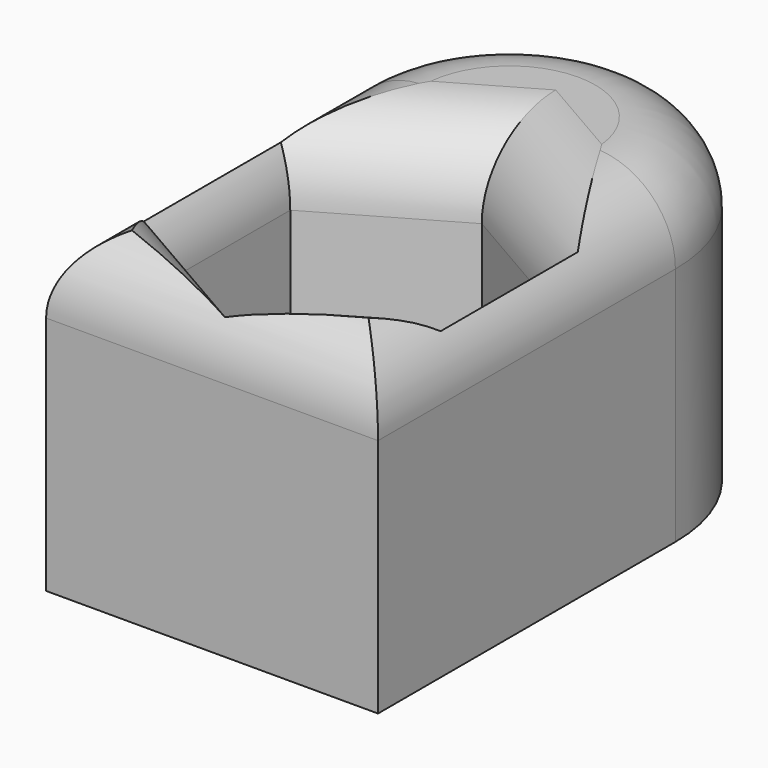
from build123d import *

# Parameters (mm, degrees)
F1_DEPTH      = 50.8
F2_T1_DEPTH   = 58.9474439621
F2_T3_DEPTH   = 52.6393949986
F2_T6_ANGLE   = 180
F2_T10_DEPTH  = 87.4865868528
F2_T16_DEPTH  = 87.4865868528
F2_T22_DEPTH  = 87.4865868528
F2_T28_DEPTH  = 87.4865868528
F2_T34_DEPTH  = 87.4865868528
F2_T40_DEPTH  = 87.4865868528
F2_T47_DEPTH  = 90.6974439621
F2_T51_DEPTH  = 84.3893949986
F2_T58_DEPTH  = 84.3893949986
F2_T62_DEPTH  = 90.6974439621
F2_T69_DEPTH  = 87.4865868528
F2_T73_DEPTH  = 87.4865868528
F2_T80_DEPTH  = 87.4865868528
F2_T84_DEPTH  = 87.4865868528
F2_T91_DEPTH  = 87.4865868528
F2_T95_DEPTH  = 87.4865868528
F2_T102_DEPTH = 87.4865868528
F2_T106_DEPTH = 87.4865868528
F2_T113_DEPTH = 87.4865868528
F2_T117_DEPTH = 87.4865868528
F2_T124_DEPTH = 87.4865868528
F2_T128_DEPTH = 87.4865868528


# Not quite as in the source:
# - a fillet or chamfer that OpenCascade refuses, or shapes differently, is made with other operations: its cross-section is extruded or revolved along the edge and cut away or added
# - a feature names something its author has since deleted; it is built from what else it names


with BuildPart() as f1:
    # F0 (on Top) → F1 (new body)
    with BuildSketch(Plane.XY):
        with BuildLine():
            Line((-26.3196974993, -29.473721981), (26.3196974993, -29.473721981))
            Line((26.3196974993, -29.473721981), (26.3196974993, 29.473721981))
            ThreePointArc((26.3196974993, 29.473721981), (0, 55.7934194803), (-26.3196974993, 29.473721981))
            Line((-26.3196974993, 29.473721981), (-26.3196974993, -29.473721981))
        make_face()
        Polygon((0, 23.9865868528), (20.7729935646, 11.9932934264), (20.7729935646, -11.9932934264), (0, -23.9865868528), (-20.7729935646, -11.9932934264), (-20.7729935646, 11.9932934264), align=None, mode=Mode.SUBTRACT)
    extrude(amount=F1_DEPTH)

    # F2: fillet of radius 12.7 on 10 edges, made by hand

    # F2_s2 → F2_t1 (cut)
    with BuildSketch(Plane.XZ.offset(-29.473721981)):
        with BuildLine():
            ThreePointArc((-26.3196974993, 38.1), (-22.5999536203, 47.0802561211), (-13.6196974993, 50.8))
            Line((-13.6196974993, 50.8), (-13.6196974993, 51.054))
            Line((-13.6196974993, 51.054), (-26.5736974993, 51.054))
            Line((-26.5736974993, 51.054), (-26.5736974993, 38.1))
            Line((-26.5736974993, 38.1), (-26.3196974993, 38.1))
        make_face()
        with BuildLine():
            ThreePointArc((26.3196974993, 38.1), (22.5999536203, 47.0802561211), (13.6196974993, 50.8))
            Line((13.6196974993, 50.8), (13.6196974993, 51.054))
            Line((13.6196974993, 51.054), (26.5736974993, 51.054))
            Line((26.5736974993, 51.054), (26.5736974993, 38.1))
            Line((26.5736974993, 38.1), (26.3196974993, 38.1))
        make_face()
    extrude(amount=F2_T1_DEPTH, mode=Mode.SUBTRACT)

    # F2_s4 → F2_t3 (cut)
    with BuildSketch(Plane.YZ.offset(-26.3196974993)):
        with BuildLine():
            ThreePointArc((-29.473721981, 38.1), (-25.7539781021, 47.0802561211), (-16.773721981, 50.8))
            Line((-16.773721981, 50.8), (-16.773721981, 51.054))
            Line((-16.773721981, 51.054), (-29.727721981, 51.054))
            Line((-29.727721981, 51.054), (-29.727721981, 38.1))
            Line((-29.727721981, 38.1), (-29.473721981, 38.1))
        make_face()
    extrude(amount=F2_T3_DEPTH, mode=Mode.SUBTRACT)

    # F2_s5 → F2_t6 (revolve, cut)
    with BuildSketch(Plane.XZ.offset(-29.473721981)):
        with BuildLine():
            ThreePointArc((26.3196974993, 38.1), (22.5999536203, 47.0802561211), (13.6196974993, 50.8))
            Line((13.6196974993, 50.8), (13.6196974993, 51.054))
            Line((13.6196974993, 51.054), (26.5736974993, 51.054))
            Line((26.5736974993, 51.054), (26.5736974993, 38.1))
            Line((26.5736974993, 38.1), (26.3196974993, 38.1))
        make_face()
    revolve(axis=Axis((0, 29.473721981, 50.8), (0, 0, 1)), revolution_arc=F2_T6_ANGLE, mode=Mode.SUBTRACT)


with BuildPart() as f2_tool8:
    # F2_s9 → F2_t10 (new body)
    with BuildSketch(Plane(origin=(-37.8828033525, -21.8716467132, 0), x_dir=(0, 0, 1), z_dir=(0.8660254038, 0.5, 0))):
        with BuildLine():
            ThreePointArc((38.1, -20.7729935646), (47.0802561211, -24.4927374435), (50.8, -33.4729935646))
            Line((50.8, -33.4729935646), (51.054, -33.4729935646))
            Line((51.054, -33.4729935646), (51.054, -20.5189935646))
            Line((51.054, -20.5189935646), (38.1, -20.5189935646))
            Line((38.1, -20.5189935646), (38.1, -20.7729935646))
        make_face()
    extrude(amount=F2_T10_DEPTH)

    split(bisect_by=Plane.YZ.offset(-20.7729935646), keep=Keep.TOP)

    split(bisect_by=Plane(origin=(10.3864967823, 17.9899401396, 0), x_dir=(0, 0, 1), z_dir=(-0.5, -0.8660254038, 0)), keep=Keep.TOP)


with BuildPart() as f1_1:
    add(f1.part)

    # F2_t7: cut F2_tool8
    add(f2_tool8.part, mode=Mode.SUBTRACT)


with BuildPart() as f2_tool14:
    # F2_s15 → F2_t16 (new body)
    with BuildSketch(Plane(origin=(-37.8828033525, 21.8716467132, 0), x_dir=(0, 0, 1), z_dir=(0.8660254038, -0.5, 0))):
        with BuildLine():
            ThreePointArc((38.1, -20.7729935646), (47.0802561211, -24.4927374435), (50.8, -33.4729935646))
            Line((50.8, -33.4729935646), (51.054, -33.4729935646))
            Line((51.054, -33.4729935646), (51.054, -20.5189935646))
            Line((51.054, -20.5189935646), (38.1, -20.5189935646))
            Line((38.1, -20.5189935646), (38.1, -20.7729935646))
        make_face()
    extrude(amount=F2_T16_DEPTH)

    split(bisect_by=Plane(origin=(-10.3864967823, 17.9899401396, 0), x_dir=(0, 0, 1), z_dir=(0.5, -0.8660254038, 0)), keep=Keep.TOP)

    split(bisect_by=Plane.YZ.offset(20.7729935646), keep=Keep.BOTTOM)


with BuildPart() as f1_2:
    add(f1_1.part)

    # F2_t13: cut F2_tool14
    add(f2_tool14.part, mode=Mode.SUBTRACT)


with BuildPart() as f2_tool20:
    # F2_s21 → F2_t22 (new body)
    with BuildSketch(Plane.XZ.offset(-43.7432934264)):
        with BuildLine():
            ThreePointArc((20.7729935646, 38.1), (24.4927374435, 47.0802561211), (33.4729935646, 50.8))
            Line((33.4729935646, 50.8), (33.4729935646, 51.054))
            Line((33.4729935646, 51.054), (20.5189935646, 51.054))
            Line((20.5189935646, 51.054), (20.5189935646, 38.1))
            Line((20.5189935646, 38.1), (20.7729935646, 38.1))
        make_face()
    extrude(amount=F2_T22_DEPTH)

    split(bisect_by=Plane(origin=(10.3864967823, 17.9899401396, 0), x_dir=(0, 0, 1), z_dir=(-0.5, -0.8660254038, 0)), keep=Keep.TOP)

    split(bisect_by=Plane(origin=(10.3864967823, -17.9899401396, 0), x_dir=(0, 0, 1), z_dir=(-0.5, 0.8660254038, 0)), keep=Keep.TOP)


with BuildPart() as f1_3:
    add(f1_2.part)

    # F2_t19: cut F2_tool20
    add(f2_tool20.part, mode=Mode.SUBTRACT)


with BuildPart() as f2_tool26:
    # F2_s27 → F2_t28 (new body)
    with BuildSketch(Plane(origin=(37.8828033525, 21.8716467132, 0), x_dir=(0, 0, 1), z_dir=(-0.8660254038, -0.5, 0))):
        with BuildLine():
            ThreePointArc((38.1, -20.7729935646), (47.0802561211, -24.4927374435), (50.8, -33.4729935646))
            Line((50.8, -33.4729935646), (51.054, -33.4729935646))
            Line((51.054, -33.4729935646), (51.054, -20.5189935646))
            Line((51.054, -20.5189935646), (38.1, -20.5189935646))
            Line((38.1, -20.5189935646), (38.1, -20.7729935646))
        make_face()
    extrude(amount=F2_T28_DEPTH)

    split(bisect_by=Plane.YZ.offset(20.7729935646), keep=Keep.BOTTOM)

    split(bisect_by=Plane(origin=(-10.3864967823, -17.9899401396, 0), x_dir=(0, 0, 1), z_dir=(0.5, 0.8660254038, 0)), keep=Keep.TOP)


with BuildPart() as f1_4:
    add(f1_3.part)

    # F2_t25: cut F2_tool26
    add(f2_tool26.part, mode=Mode.SUBTRACT)


with BuildPart() as f2_tool32:
    # F2_s33 → F2_t34 (new body)
    with BuildSketch(Plane(origin=(37.8828033525, -21.8716467132, 0), x_dir=(0, 0, 1), z_dir=(-0.8660254038, 0.5, 0))):
        with BuildLine():
            ThreePointArc((38.1, -20.7729935646), (47.0802561211, -24.4927374435), (50.8, -33.4729935646))
            Line((50.8, -33.4729935646), (51.054, -33.4729935646))
            Line((51.054, -33.4729935646), (51.054, -20.5189935646))
            Line((51.054, -20.5189935646), (38.1, -20.5189935646))
            Line((38.1, -20.5189935646), (38.1, -20.7729935646))
        make_face()
    extrude(amount=F2_T34_DEPTH)

    split(bisect_by=Plane(origin=(10.3864967823, -17.9899401396, 0), x_dir=(0, 0, 1), z_dir=(-0.5, 0.8660254038, 0)), keep=Keep.TOP)

    split(bisect_by=Plane.YZ.offset(-20.7729935646), keep=Keep.TOP)


with BuildPart() as f1_5:
    add(f1_4.part)

    # F2_t31: cut F2_tool32
    add(f2_tool32.part, mode=Mode.SUBTRACT)


with BuildPart() as f2_tool38:
    # F2_s39 → F2_t40 (new body)
    with BuildSketch(Plane.XZ.offset(43.7432934264)):
        with BuildLine():
            ThreePointArc((-20.7729935646, 38.1), (-24.4927374435, 47.0802561211), (-33.4729935646, 50.8))
            Line((-33.4729935646, 50.8), (-33.4729935646, 51.054))
            Line((-33.4729935646, 51.054), (-20.5189935646, 51.054))
            Line((-20.5189935646, 51.054), (-20.5189935646, 38.1))
            Line((-20.5189935646, 38.1), (-20.7729935646, 38.1))
        make_face()
    extrude(amount=-F2_T40_DEPTH)

    split(bisect_by=Plane(origin=(-10.3864967823, 17.9899401396, 0), x_dir=(0, 0, 1), z_dir=(0.5, -0.8660254038, 0)), keep=Keep.TOP)

    split(bisect_by=Plane(origin=(-10.3864967823, -17.9899401396, 0), x_dir=(0, 0, 1), z_dir=(0.5, 0.8660254038, 0)), keep=Keep.TOP)


with BuildPart() as f1_6:
    add(f1_5.part)

    # F2_t37: cut F2_tool38
    add(f2_tool38.part, mode=Mode.SUBTRACT)


with BuildPart() as f2_tool45:
    # F2_s46 → F2_t47 (new body)
    with BuildSketch(Plane.XZ.offset(-29.473721981)):
        with BuildLine():
            ThreePointArc((-26.3196974993, 38.1), (-22.5999536203, 47.0802561211), (-13.6196974993, 50.8))
            Line((-13.6196974993, 50.8), (-13.6196974993, 51.054))
            Line((-13.6196974993, 51.054), (-26.5736974993, 51.054))
            Line((-26.5736974993, 51.054), (-26.5736974993, 38.1))
            Line((-26.5736974993, 38.1), (-26.3196974993, 38.1))
        make_face()
    extrude(amount=F2_T47_DEPTH)

    split(bisect_by=Plane.XZ.offset(29.473721981), keep=Keep.TOP)


with BuildPart() as f2_tool49:
    # F2_s50 → F2_t51 (new body)
    with BuildSketch(Plane.YZ.offset(-58.0696974993)):
        with BuildLine():
            ThreePointArc((-29.473721981, 38.1), (-25.7539781021, 47.0802561211), (-16.773721981, 50.8))
            Line((-16.773721981, 50.8), (-16.773721981, 51.054))
            Line((-16.773721981, 51.054), (-29.727721981, 51.054))
            Line((-29.727721981, 51.054), (-29.727721981, 38.1))
            Line((-29.727721981, 38.1), (-29.473721981, 38.1))
        make_face()
    extrude(amount=F2_T51_DEPTH)

    split(bisect_by=Plane.YZ.offset(-26.3196974993), keep=Keep.BOTTOM)


with BuildPart() as f2_tool45_1:
    add(f2_tool45.part)

    # F2_t53: intersect F2_tool49
    add(f2_tool49.part, mode=Mode.INTERSECT)


with BuildPart() as f1_7:
    add(f1_6.part)

    # F2_t43: cut F2_tool45
    add(f2_tool45_1.part, mode=Mode.SUBTRACT)


with BuildPart() as f2_tool56:
    # F2_s57 → F2_t58 (new body)
    with BuildSketch(Plane.YZ.offset(-26.3196974993)):
        with BuildLine():
            ThreePointArc((-29.473721981, 38.1), (-25.7539781021, 47.0802561211), (-16.773721981, 50.8))
            Line((-16.773721981, 50.8), (-16.773721981, 51.054))
            Line((-16.773721981, 51.054), (-29.727721981, 51.054))
            Line((-29.727721981, 51.054), (-29.727721981, 38.1))
            Line((-29.727721981, 38.1), (-29.473721981, 38.1))
        make_face()
    extrude(amount=F2_T58_DEPTH)

    split(bisect_by=Plane.YZ.offset(26.3196974993), keep=Keep.TOP)


with BuildPart() as f2_tool60:
    # F2_s61 → F2_t62 (new body)
    with BuildSketch(Plane.XZ.offset(61.223721981)):
        with BuildLine():
            ThreePointArc((26.3196974993, 38.1), (22.5999536203, 47.0802561211), (13.6196974993, 50.8))
            Line((13.6196974993, 50.8), (13.6196974993, 51.054))
            Line((13.6196974993, 51.054), (26.5736974993, 51.054))
            Line((26.5736974993, 51.054), (26.5736974993, 38.1))
            Line((26.5736974993, 38.1), (26.3196974993, 38.1))
        make_face()
    extrude(amount=-F2_T62_DEPTH)

    split(bisect_by=Plane.XZ.offset(29.473721981), keep=Keep.TOP)


with BuildPart() as f2_tool56_1:
    add(f2_tool56.part)

    # F2_t64: intersect F2_tool60
    add(f2_tool60.part, mode=Mode.INTERSECT)


with BuildPart() as f1_8:
    add(f1_7.part)

    # F2_t54: cut F2_tool56
    add(f2_tool56_1.part, mode=Mode.SUBTRACT)


with BuildPart() as f2_tool67:
    # F2_s68 → F2_t69 (new body)
    with BuildSketch(Plane(origin=(-37.8828033525, -21.8716467132, 0), x_dir=(0, 0, 1), z_dir=(0.8660254038, 0.5, 0))):
        with BuildLine():
            ThreePointArc((38.1, -20.7729935646), (47.0802561211, -24.4927374435), (50.8, -33.4729935646))
            Line((50.8, -33.4729935646), (51.054, -33.4729935646))
            Line((51.054, -33.4729935646), (51.054, -20.5189935646))
            Line((51.054, -20.5189935646), (38.1, -20.5189935646))
            Line((38.1, -20.5189935646), (38.1, -20.7729935646))
        make_face()
    extrude(amount=F2_T69_DEPTH)

    split(bisect_by=Plane.YZ.offset(-20.7729935646), keep=Keep.BOTTOM)


with BuildPart() as f2_tool71:
    # F2_s72 → F2_t73 (new body)
    with BuildSketch(Plane.XZ.offset(43.7432934264)):
        with BuildLine():
            ThreePointArc((-20.7729935646, 38.1), (-24.4927374435, 47.0802561211), (-33.4729935646, 50.8))
            Line((-33.4729935646, 50.8), (-33.4729935646, 51.054))
            Line((-33.4729935646, 51.054), (-20.5189935646, 51.054))
            Line((-20.5189935646, 51.054), (-20.5189935646, 38.1))
            Line((-20.5189935646, 38.1), (-20.7729935646, 38.1))
        make_face()
    extrude(amount=-F2_T73_DEPTH)

    split(bisect_by=Plane(origin=(-10.3864967823, 17.9899401396, 0), x_dir=(0, 0, 1), z_dir=(-0.5, 0.8660254038, 0)), keep=Keep.TOP)


with BuildPart() as f2_tool67_1:
    add(f2_tool67.part)

    # F2_t75: intersect F2_tool71
    add(f2_tool71.part, mode=Mode.INTERSECT)


with BuildPart() as f1_9:
    add(f1_8.part)

    # F2_t65: cut F2_tool67
    add(f2_tool67_1.part, mode=Mode.SUBTRACT)


with BuildPart() as f2_tool78:
    # F2_s79 → F2_t80 (new body)
    with BuildSketch(Plane(origin=(-37.8828033525, -21.8716467132, 0), x_dir=(0, 0, 1), z_dir=(0.8660254038, 0.5, 0))):
        with BuildLine():
            ThreePointArc((38.1, -20.7729935646), (47.0802561211, -24.4927374435), (50.8, -33.4729935646))
            Line((50.8, -33.4729935646), (51.054, -33.4729935646))
            Line((51.054, -33.4729935646), (51.054, -20.5189935646))
            Line((51.054, -20.5189935646), (38.1, -20.5189935646))
            Line((38.1, -20.5189935646), (38.1, -20.7729935646))
        make_face()
    extrude(amount=F2_T80_DEPTH)

    split(bisect_by=Plane(origin=(10.3864967823, 17.9899401396, 0), x_dir=(0, 0, 1), z_dir=(0.5, 0.8660254038, 0)), keep=Keep.TOP)


with BuildPart() as f2_tool82:
    # F2_s83 → F2_t84 (new body)
    with BuildSketch(Plane(origin=(-37.8828033525, 21.8716467132, 0), x_dir=(0, 0, 1), z_dir=(0.8660254038, -0.5, 0))):
        with BuildLine():
            ThreePointArc((38.1, -20.7729935646), (47.0802561211, -24.4927374435), (50.8, -33.4729935646))
            Line((50.8, -33.4729935646), (51.054, -33.4729935646))
            Line((51.054, -33.4729935646), (51.054, -20.5189935646))
            Line((51.054, -20.5189935646), (38.1, -20.5189935646))
            Line((38.1, -20.5189935646), (38.1, -20.7729935646))
        make_face()
    extrude(amount=F2_T84_DEPTH)

    split(bisect_by=Plane(origin=(-10.3864967823, 17.9899401396, 0), x_dir=(0, 0, 1), z_dir=(-0.5, 0.8660254038, 0)), keep=Keep.TOP)


with BuildPart() as f2_tool78_1:
    add(f2_tool78.part)

    # F2_t86: intersect F2_tool82
    add(f2_tool82.part, mode=Mode.INTERSECT)


with BuildPart() as f1_10:
    add(f1_9.part)

    # F2_t76: cut F2_tool78
    add(f2_tool78_1.part, mode=Mode.SUBTRACT)


with BuildPart() as f2_tool89:
    # F2_s90 → F2_t91 (new body)
    with BuildSketch(Plane(origin=(-37.8828033525, 21.8716467132, 0), x_dir=(0, 0, 1), z_dir=(0.8660254038, -0.5, 0))):
        with BuildLine():
            ThreePointArc((38.1, -20.7729935646), (47.0802561211, -24.4927374435), (50.8, -33.4729935646))
            Line((50.8, -33.4729935646), (51.054, -33.4729935646))
            Line((51.054, -33.4729935646), (51.054, -20.5189935646))
            Line((51.054, -20.5189935646), (38.1, -20.5189935646))
            Line((38.1, -20.5189935646), (38.1, -20.7729935646))
        make_face()
    extrude(amount=F2_T91_DEPTH)

    split(bisect_by=Plane.YZ.offset(20.7729935646), keep=Keep.TOP)


with BuildPart() as f2_tool93:
    # F2_s94 → F2_t95 (new body)
    with BuildSketch(Plane.XZ.offset(-43.7432934264)):
        with BuildLine():
            ThreePointArc((20.7729935646, 38.1), (24.4927374435, 47.0802561211), (33.4729935646, 50.8))
            Line((33.4729935646, 50.8), (33.4729935646, 51.054))
            Line((33.4729935646, 51.054), (20.5189935646, 51.054))
            Line((20.5189935646, 51.054), (20.5189935646, 38.1))
            Line((20.5189935646, 38.1), (20.7729935646, 38.1))
        make_face()
    extrude(amount=F2_T95_DEPTH)

    split(bisect_by=Plane(origin=(10.3864967823, 17.9899401396, 0), x_dir=(0, 0, 1), z_dir=(0.5, 0.8660254038, 0)), keep=Keep.TOP)


with BuildPart() as f2_tool89_1:
    add(f2_tool89.part)

    # F2_t97: intersect F2_tool93
    add(f2_tool93.part, mode=Mode.INTERSECT)


with BuildPart() as f1_11:
    add(f1_10.part)

    # F2_t87: cut F2_tool89
    add(f2_tool89_1.part, mode=Mode.SUBTRACT)


with BuildPart() as f2_tool100:
    # F2_s101 → F2_t102 (new body)
    with BuildSketch(Plane.XZ.offset(-43.7432934264)):
        with BuildLine():
            ThreePointArc((20.7729935646, 38.1), (24.4927374435, 47.0802561211), (33.4729935646, 50.8))
            Line((33.4729935646, 50.8), (33.4729935646, 51.054))
            Line((33.4729935646, 51.054), (20.5189935646, 51.054))
            Line((20.5189935646, 51.054), (20.5189935646, 38.1))
            Line((20.5189935646, 38.1), (20.7729935646, 38.1))
        make_face()
    extrude(amount=F2_T102_DEPTH)

    split(bisect_by=Plane(origin=(10.3864967823, -17.9899401396, 0), x_dir=(0, 0, 1), z_dir=(0.5, -0.8660254038, 0)), keep=Keep.TOP)


with BuildPart() as f2_tool104:
    # F2_s105 → F2_t106 (new body)
    with BuildSketch(Plane(origin=(37.8828033525, 21.8716467132, 0), x_dir=(0, 0, 1), z_dir=(-0.8660254038, -0.5, 0))):
        with BuildLine():
            ThreePointArc((38.1, -20.7729935646), (47.0802561211, -24.4927374435), (50.8, -33.4729935646))
            Line((50.8, -33.4729935646), (51.054, -33.4729935646))
            Line((51.054, -33.4729935646), (51.054, -20.5189935646))
            Line((51.054, -20.5189935646), (38.1, -20.5189935646))
            Line((38.1, -20.5189935646), (38.1, -20.7729935646))
        make_face()
    extrude(amount=F2_T106_DEPTH)

    split(bisect_by=Plane.YZ.offset(20.7729935646), keep=Keep.TOP)


with BuildPart() as f2_tool100_1:
    add(f2_tool100.part)

    # F2_t108: intersect F2_tool104
    add(f2_tool104.part, mode=Mode.INTERSECT)


with BuildPart() as f1_12:
    add(f1_11.part)

    # F2_t98: cut F2_tool100
    add(f2_tool100_1.part, mode=Mode.SUBTRACT)


with BuildPart() as f2_tool111:
    # F2_s112 → F2_t113 (new body)
    with BuildSketch(Plane(origin=(37.8828033525, 21.8716467132, 0), x_dir=(0, 0, 1), z_dir=(-0.8660254038, -0.5, 0))):
        with BuildLine():
            ThreePointArc((38.1, -20.7729935646), (47.0802561211, -24.4927374435), (50.8, -33.4729935646))
            Line((50.8, -33.4729935646), (51.054, -33.4729935646))
            Line((51.054, -33.4729935646), (51.054, -20.5189935646))
            Line((51.054, -20.5189935646), (38.1, -20.5189935646))
            Line((38.1, -20.5189935646), (38.1, -20.7729935646))
        make_face()
    extrude(amount=F2_T113_DEPTH)

    split(bisect_by=Plane(origin=(-10.3864967823, -17.9899401396, 0), x_dir=(0, 0, 1), z_dir=(-0.5, -0.8660254038, 0)), keep=Keep.TOP)


with BuildPart() as f2_tool115:
    # F2_s116 → F2_t117 (new body)
    with BuildSketch(Plane(origin=(37.8828033525, -21.8716467132, 0), x_dir=(0, 0, 1), z_dir=(-0.8660254038, 0.5, 0))):
        with BuildLine():
            ThreePointArc((38.1, -20.7729935646), (47.0802561211, -24.4927374435), (50.8, -33.4729935646))
            Line((50.8, -33.4729935646), (51.054, -33.4729935646))
            Line((51.054, -33.4729935646), (51.054, -20.5189935646))
            Line((51.054, -20.5189935646), (38.1, -20.5189935646))
            Line((38.1, -20.5189935646), (38.1, -20.7729935646))
        make_face()
    extrude(amount=F2_T117_DEPTH)

    split(bisect_by=Plane(origin=(10.3864967823, -17.9899401396, 0), x_dir=(0, 0, 1), z_dir=(0.5, -0.8660254038, 0)), keep=Keep.TOP)


with BuildPart() as f2_tool111_1:
    add(f2_tool111.part)

    # F2_t119: intersect F2_tool115
    add(f2_tool115.part, mode=Mode.INTERSECT)


with BuildPart() as f1_13:
    add(f1_12.part)

    # F2_t109: cut F2_tool111
    add(f2_tool111_1.part, mode=Mode.SUBTRACT)


with BuildPart() as f2_tool122:
    # F2_s123 → F2_t124 (new body)
    with BuildSketch(Plane(origin=(37.8828033525, -21.8716467132, 0), x_dir=(0, 0, 1), z_dir=(-0.8660254038, 0.5, 0))):
        with BuildLine():
            ThreePointArc((38.1, -20.7729935646), (47.0802561211, -24.4927374435), (50.8, -33.4729935646))
            Line((50.8, -33.4729935646), (51.054, -33.4729935646))
            Line((51.054, -33.4729935646), (51.054, -20.5189935646))
            Line((51.054, -20.5189935646), (38.1, -20.5189935646))
            Line((38.1, -20.5189935646), (38.1, -20.7729935646))
        make_face()
    extrude(amount=F2_T124_DEPTH)

    split(bisect_by=Plane.YZ.offset(-20.7729935646), keep=Keep.BOTTOM)


with BuildPart() as f2_tool126:
    # F2_s127 → F2_t128 (new body)
    with BuildSketch(Plane.XZ.offset(43.7432934264)):
        with BuildLine():
            ThreePointArc((-20.7729935646, 38.1), (-24.4927374435, 47.0802561211), (-33.4729935646, 50.8))
            Line((-33.4729935646, 50.8), (-33.4729935646, 51.054))
            Line((-33.4729935646, 51.054), (-20.5189935646, 51.054))
            Line((-20.5189935646, 51.054), (-20.5189935646, 38.1))
            Line((-20.5189935646, 38.1), (-20.7729935646, 38.1))
        make_face()
    extrude(amount=-F2_T128_DEPTH)

    split(bisect_by=Plane(origin=(-10.3864967823, -17.9899401396, 0), x_dir=(0, 0, 1), z_dir=(-0.5, -0.8660254038, 0)), keep=Keep.TOP)


with BuildPart() as f2_tool122_1:
    add(f2_tool122.part)

    # F2_t130: intersect F2_tool126
    add(f2_tool126.part, mode=Mode.INTERSECT)


with BuildPart() as f1_14:
    add(f1_13.part)

    # F2_t120: cut F2_tool122
    add(f2_tool122_1.part, mode=Mode.SUBTRACT)


solid = f1_14.part
